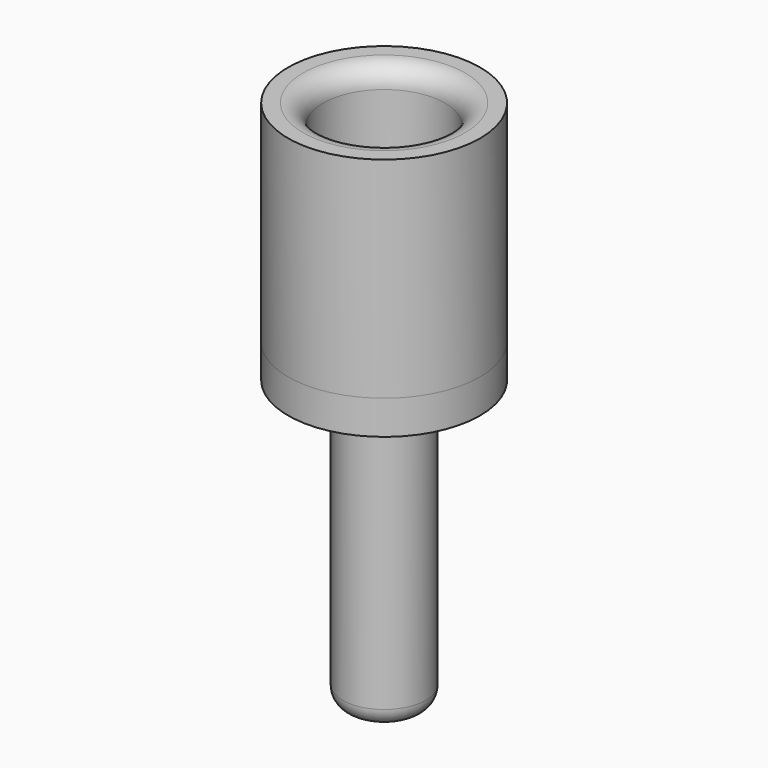
from build123d import *

# Parameters (mm, degrees)
F0_R     = 1.5625
F0_R_2   = 0.9875
F1_DEPTH = 12
F2_R     = 3.6
F2_R_2   = 2.5
F2_R_3   = 1.5625
F3_DEPTH = 1.275
F4_R     = 3.6
F4_R_2   = 2.2875
F5_DEPTH = 7.875
F6_R     = 2.2875
F6_R_2   = 1.115
F7_DEPTH = 2
F9_R     = 0.75
F11_R    = 0.1279533188


# Not quite as in the source:
# - a fillet or chamfer that OpenCascade refuses, or shapes differently, is made with other operations: its cross-section is extruded or revolved along the edge and cut away or added


with BuildPart() as f1:
    # F0 (on Top) → F1 (new body)
    with BuildSketch(Plane.XY):
        Circle(F0_R)
        Circle(F0_R_2, mode=Mode.SUBTRACT)
    extrude(amount=-F1_DEPTH)

    # F2 (on face) → F3 (join)
    with BuildSketch(Plane.XY):
        Circle(F2_R)
        Circle(F2_R_2, mode=Mode.SUBTRACT)
        Circle(F2_R_2)
        Circle(F2_R_3, mode=Mode.SUBTRACT)
    extrude(amount=-F3_DEPTH)

    # F10: fillet of radius 0.6759797975 on 1 edges, made by hand

    # F10_s1 → F10_t2 (revolve, cut)
    with BuildSketch(Plane.XZ):
        with BuildLine():
            ThreePointArc((1.5625, -11.3316050815), (1.3989697072, -11.7724499428), (0.9875, -12))
            Line((0.9875, -12), (1.5625, -12))
            Line((1.5625, -12), (1.5625, -11.3316050815))
        make_face()
    revolve(axis=Axis((0, 0, -12), (0, 0, 1)), mode=Mode.SUBTRACT)

    # F11
    f11_edges = [f1.edges().sort_by_distance(p)[0] for p in [
        (-0.9875, 0, 0),
    ]]
    fillet(f11_edges, radius=F11_R)


with BuildPart() as f5:
    # F4 (on face) → F5 (new body)
    with BuildSketch(Plane.XY):
        Circle(F4_R)
        Circle(F4_R_2, mode=Mode.SUBTRACT)
    extrude(amount=F5_DEPTH)

    # F6 (on face) → F7 (join)
    with BuildSketch(Plane(origin=(0, 0, 0), x_dir=(1, 0, 0), z_dir=(0, 0, -1))):
        Circle(F6_R)
        Circle(F6_R_2, mode=Mode.SUBTRACT)
    extrude(amount=-F7_DEPTH)

    # F8: fillet of radius 1.75 on 1 edges, made by hand

    # F8_s1 → F8_t2 (revolve, cut)
    with BuildSketch(Plane.XZ):
        with BuildLine():
            ThreePointArc((1.115, 0.348033369), (1.4379181873, 1.360919098), (2.2875, 2))
            Line((2.2875, 2), (1.115, 2))
            Line((1.115, 2), (1.115, 0.348033369))
        make_face()
    revolve(axis=Axis((0, 0, 2), (0, 0, -1)), mode=Mode.SUBTRACT)

    # F9
    f9_edges = [f5.edges().sort_by_distance(p)[0] for p in [
        (-2.2875, 0, 7.875),
    ]]
    fillet(f9_edges, radius=F9_R)


solid = Compound([f1.part, f5.part])
